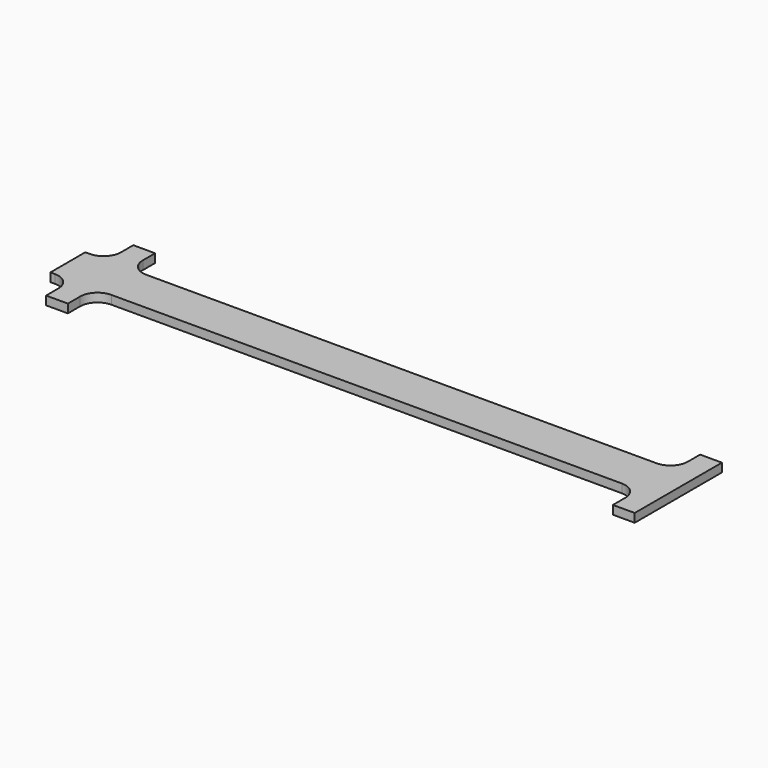
from build123d import *

# Parameters (mm, degrees)
F1_DEPTH = 0.79375


# Not quite as in the source:
# - a length typed as a fraction of an inch, garbled in the dataset ("3 / 203.2 mm" for 3/8 in), is restored


with BuildPart() as f1:
    # F0 (on Top) → F1 (new body)
    with BuildSketch(Plane.XY):
        with BuildLine():
            ThreePointArc((0, 3.5875), (-0.4649679849, 2.4649679849), (-1.5875, 2))
            Line((-1.5875, 2), (-48.4125, 2))
            ThreePointArc((-48.4125, 2), (-49.5350320151, 2.4649679849), (-50, 3.5875))
            Line((-50, 3.5875), (-50, 5))
            Line((-50, 5), (-52, 5))
            Line((-52, 5), (-52, 3.5875))
            ThreePointArc((-52, 3.5875), (-52.4649679849, 2.4649679849), (-53.5875, 2))
            Line((-53.5875, 2), (-54, 2))
            Line((-54, 2), (-54, -2))
            Line((-54, -2), (-53.5875, -2))
            ThreePointArc((-53.5875, -2), (-52.4649679849, -2.4649679849), (-52, -3.5875))
            Line((-52, -3.5875), (-52, -5))
            Line((-52, -5), (-50, -5))
            Line((-50, -5), (-50, -3.5875))
            ThreePointArc((-50, -3.5875), (-49.5350320151, -2.4649679849), (-48.4125, -2))
            Line((-48.4125, -2), (-1.5875, -2))
            ThreePointArc((-1.5875, -2), (-0.4649679849, -2.4649679849), (0, -3.5875))
            Line((0, -3.5875), (0, -5))
            Line((0, -5), (2, -5))
            Line((2, -5), (2, 5))
            Line((2, 5), (0, 5))
            Line((0, 5), (0, 3.5875))
        make_face()
    extrude(amount=F1_DEPTH)


solid = f1.part
